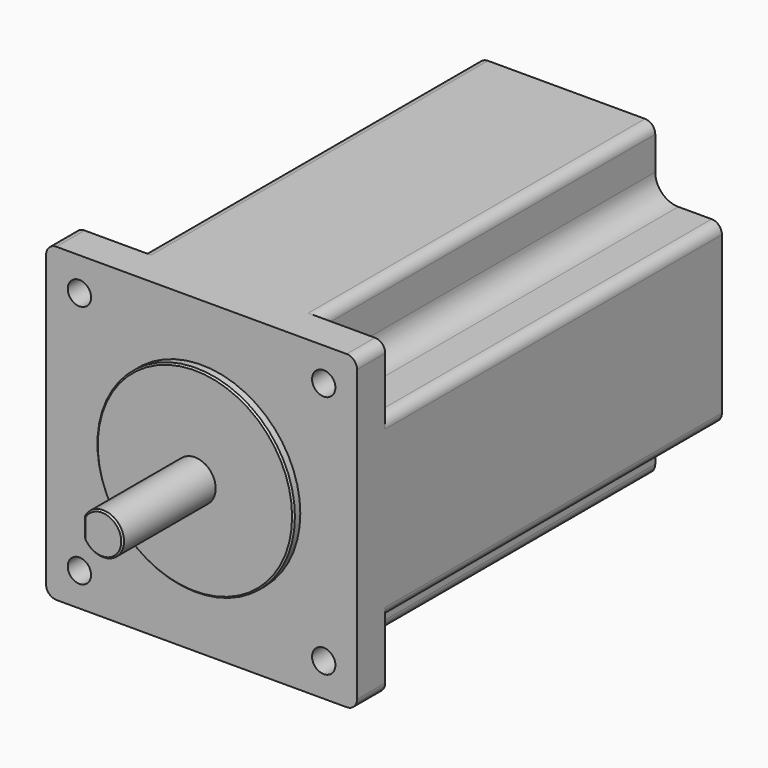
from build123d import *

# Parameters (mm, degrees)
F0_W     = 12.86
F0_H     = 12.86
F0_R     = 2.25
F0_R_2   = 19.05
F1_DEPTH = 6.8
F2_DEPTH = 1.6
F3_DEPTH = 88
F4_R     = 4.45
F5_R     = 2
F6_DEPTH = 10
F7_DEPTH = 24
F8_DEPTH = 103
F9_SIZE  = 0.3


with BuildPart() as f1:
    # F0 (on Front) → F1 (new body)
    with BuildSketch(Plane.XZ):
        with Locations((23.57, -23.57)):
            Rectangle(F0_W, F0_H)
        with Locations((23.57, -23.57)):
            Circle(F0_R, mode=Mode.SUBTRACT)
        Polygon((-17.14, -30), (17.14, -30), (17.14, -17.14), (30, -17.14), (30, 17.14), (17.14, 17.14), (17.14, 30), (-17.14, 30), (-17.14, 17.14), (-30, 17.14), (-30, -17.14), (-17.14, -17.14), align=None)
        Circle(F0_R_2, mode=Mode.SUBTRACT)
        with Locations((-23.57, -23.57)):
            Rectangle(F0_W, F0_H)
        with Locations((-23.57, -23.57)):
            Circle(F0_R, mode=Mode.SUBTRACT)
        with Locations((23.57, 23.57)):
            Rectangle(F0_W, F0_H)
        with Locations((23.57, 23.57)):
            Circle(F0_R, mode=Mode.SUBTRACT)
        with Locations((-23.57, 23.57)):
            Rectangle(F0_W, F0_H)
        with Locations((-23.57, 23.57)):
            Circle(F0_R, mode=Mode.SUBTRACT)
        Circle(F0_R_2)
        with BuildLine():
            ThreePointArc((-3.5, 1.9364916731), (1, 3.8729833462), (4, 0))
            ThreePointArc((4, 0), (1, -3.8729833462), (-3.5, -1.9364916731))
            ThreePointArc((-3.5, -1.9364916731), (-4, 0), (-3.5, 1.9364916731))
        make_face(mode=Mode.SUBTRACT)
    extrude(amount=-F1_DEPTH)

    # F0 (on Front) → F2 (join)
    with BuildSketch(Plane.XZ):
        Circle(F0_R_2)
        with BuildLine():
            ThreePointArc((-3.5, 1.9364916731), (1, 3.8729833462), (4, 0))
            ThreePointArc((4, 0), (1, -3.8729833462), (-3.5, -1.9364916731))
            ThreePointArc((-3.5, -1.9364916731), (-4, 0), (-3.5, 1.9364916731))
        make_face(mode=Mode.SUBTRACT)
    extrude(amount=F2_DEPTH)

    # F0 (on Front) → F3 (join)
    with BuildSketch(Plane.XZ):
        Polygon((-17.14, -30), (17.14, -30), (17.14, -17.14), (30, -17.14), (30, 17.14), (17.14, 17.14), (17.14, 30), (-17.14, 30), (-17.14, 17.14), (-30, 17.14), (-30, -17.14), (-17.14, -17.14), align=None)
        Circle(F0_R_2, mode=Mode.SUBTRACT)
        Circle(F0_R_2)
        with BuildLine():
            ThreePointArc((-3.5, 1.9364916731), (1, 3.8729833462), (4, 0))
            ThreePointArc((4, 0), (1, -3.8729833462), (-3.5, -1.9364916731))
            ThreePointArc((-3.5, -1.9364916731), (-4, 0), (-3.5, 1.9364916731))
        make_face(mode=Mode.SUBTRACT)
    extrude(amount=-F3_DEPTH)

    # F4
    f4_edges = [f1.edges().sort_by_distance(p)[0] for p in [
        (17.14, 47.4, 17.14),
        (17.14, 47.4, -17.14),
        (-17.14, 47.4, 17.14),
        (-17.14, 47.4, -17.14),
    ]]
    fillet(f4_edges, radius=F4_R)

    # F5
    f5_edges = [f1.edges().sort_by_distance(p)[0] for p in [
        (-30, 3.4, 30),
        (30, 3.4, 30),
        (-17.14, 47.4, 30),
        (-30, 47.4, 17.14),
        (17.14, 47.4, 30),
        (-30, 3.4, -30),
        (30, 3.4, -30),
        (30, 47.4, 17.14),
        (30, 47.4, -17.14),
        (17.14, 47.4, -30),
        (-17.14, 47.4, -30),
        (-30, 47.4, -17.14),
    ]]
    fillet(f5_edges, radius=F5_R)

    # F0 (on Front) → F6 (join)
    with BuildSketch(Plane.XZ):
        with BuildLine():
            Line((-3.5, -1.9364916731), (-3.5, 1.9364916731))
            ThreePointArc((-3.5, 1.9364916731), (-4, 0), (-3.5, -1.9364916731))
        make_face()
    extrude(amount=F6_DEPTH)

    # F0 (on Front) → F7 (join)
    with BuildSketch(Plane.XZ):
        with BuildLine():
            ThreePointArc((-3.5, -1.9364916731), (1, -3.8729833462), (4, 0))
            ThreePointArc((4, 0), (1, 3.8729833462), (-3.5, 1.9364916731))
            Line((-3.5, 1.9364916731), (-3.5, -1.9364916731))
        make_face()
    extrude(amount=F7_DEPTH)

    # F0 (on Front) → F8 (join)
    with BuildSketch(Plane.XZ):
        with BuildLine():
            ThreePointArc((-3.5, -1.9364916731), (1, -3.8729833462), (4, 0))
            ThreePointArc((4, 0), (1, 3.8729833462), (-3.5, 1.9364916731))
            Line((-3.5, 1.9364916731), (-3.5, -1.9364916731))
        make_face()
    extrude(amount=-F8_DEPTH)

    # F9
    f9_edges = [f1.edges().sort_by_distance(p)[0] for p in [
        (4, -24, 0),
        (-3.5, -24, 0),
        (-19.05, -1.6, 0),
    ]]
    chamfer(f9_edges, length=F9_SIZE)


solid = f1.part
